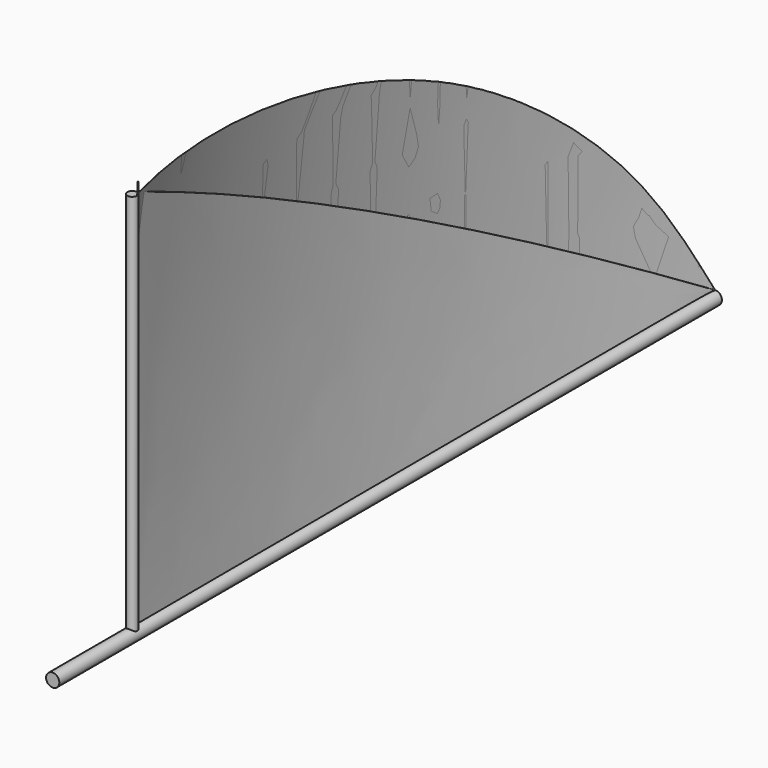
from build123d import *

# Parameters (mm, degrees)
F0_R      = 50
F1_DEPTH  = 6250
F3_DEPTH  = 2925
F8_ANGLE  = 12
F10_DEPTH = 4665.44235
F14_W     = 1
F14_H     = 5462.5


# Not quite as in the source:
# - the program builds the solid bodies; features that only make, move or delete a surface that nothing else refers to are left out


with BuildPart() as f1:
    # F0 (on Front) → F1 (new body)
    with BuildSketch(Plane.XZ):
        Circle(F0_R)
    extrude(amount=-F1_DEPTH)

    # F2 (on Top) → F3 (join)
    with BuildSketch(Plane.XY):
        with BuildLine():
            Line((37.5, 750), (0, 750))
            Line((0, 750), (-37.5, 750))
            ThreePointArc((-37.5, 750), (0, 712.5), (37.5, 750))
        make_face()
        with BuildLine():
            Line((-37.5, 750), (0, 750))
            Line((0, 750), (37.5, 750))
            ThreePointArc((37.5, 750), (0, 787.5), (-37.5, 750))
        make_face()
    extrude(amount=F3_DEPTH)


with BuildPart() as f8:
    # F4 (on Top) → F8 (revolve)
    with BuildSketch(Plane.XY):
        with BuildLine():
            ThreePointArc((0, 750), (-524.4069061533, 3500), (0, 6250))
            Line((0, 6250), (-1.0754611694, 6250))
            ThreePointArc((-1.0754611694, 6250), (-525.4069061533, 3500), (-1.0754611694, 750))
            Line((-1.0754611694, 750), (0, 750))
        make_face()
    revolve(axis=Axis((43735.8984947205, -12797.8763580322, 1000), (-0.1809418839, 0.9834937898, 0)), revolution_arc=F8_ANGLE)

    # F9 (on Right) → F10 (cut, symmetric)
    with BuildSketch(Plane.YZ):
        with BuildLine():
            add(Edge.make_bspline(
                [(6250, 50), (6096.3560088411, 363.6275828034), (5741.7081245527, 1087.5566987858), (4182.6394026515, 2380.8782608117), (2030.1958188897, 2725.8394560388), (787.5, 2925)],
                knots=[0, 0, 0, 0, 0.2441836637, 0.5636355777, 1, 1, 1, 1], degree=3))
            Line((6250, 50), (32368.7057495117, 50))
            Line((32368.7057495117, 50), (29612.3161315918, 45971.3554382324))
            Line((29612.3161315918, 45971.3554382324), (-10598.4106063843, 45971.3554382324))
            Line((-10598.4106063843, 45971.3554382324), (787.5, 2925))
        make_face()
    extrude(amount=F10_DEPTH, both=True, mode=Mode.SUBTRACT)


with BuildPart() as f15:
    # F14 (on Top) → F15 section 0
    with BuildSketch(Plane.XY):
        with Locations((-0.5, 3518.75)):
            Rectangle(F14_W, F14_H)
    # F13 (on line) → F15 section 1
    with BuildSketch(Plane(origin=(738.7902790807, 1284.1573955545, 2439.8990515535), x_dir=(0.9659258263, -0.120544047, -0.2290336893), z_dir=(0.2588190451, 0.449876508, 0.8547653652))):
        with BuildLine():
            ThreePointArc((-764.8519782508, -665.4352159096), (-1055.1936187444, 2421.0081761681), (-764.8519782508, 5507.4515682458))
            Line((-764.8519782508, 5507.4515682458), (-765.8698334753, 5507.4515682458))
            ThreePointArc((-765.8698334753, 5507.4515682458), (-1056.1936187444, 2421.0081761681), (-765.8698334753, -665.4352159096))
            Line((-765.8698334753, -665.4352159096), (-764.8519782508, -665.4352159096))
        make_face()
    loft()


solid = Compound([f1.part, f8.part, f15.part])
